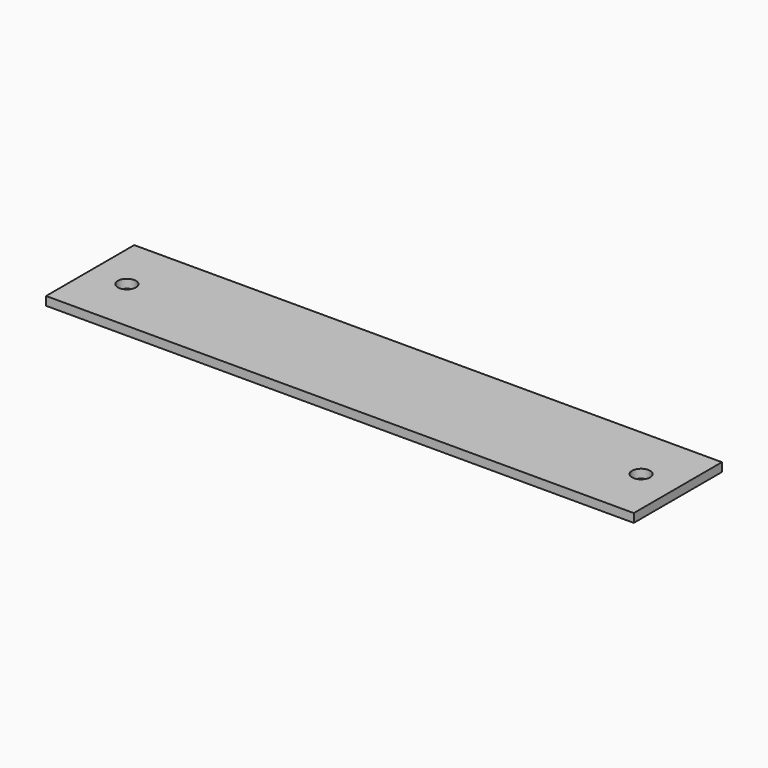
from build123d import *

# Parameters (mm, degrees)
F1_DEPTH = 3


with BuildPart() as f1:
    # F0 (on Top) → F1 (new body)
    with BuildSketch(Plane.XY):
        with BuildLine():
            Line((95.9196680397, 3.7129714398), (-5.6803319603, 3.7129714398))
            Line((-5.6803319603, 3.7129714398), (-5.6803319603, -15.3370285602))
            Line((-5.6803319603, -15.3370285602), (45.1196680397, -15.3370285602))
            Line((45.1196680397, -15.3370285602), (70.5196680397, -15.3370285602))
            Line((70.5196680397, -15.3370285602), (80.0952486641, -15.3370285602))
            ThreePointArc((80.0952486641, -15.3370285602), (83.2196680397, -12.2126091846), (86.3440874153, -15.3370285602))
            Line((86.3440874153, -15.3370285602), (95.9196680397, -15.3370285602))
            Line((95.9196680397, -15.3370285602), (95.9196680397, 3.7129714398))
        make_face()
        with BuildLine():
            Line((-97.7047513359, -15.3370285602), (-107.2803319603, -15.3370285602))
            Line((-107.2803319603, -15.3370285602), (-107.2803319603, -34.3870285602))
            Line((-107.2803319603, -34.3870285602), (-5.6803319603, -34.3870285602))
            Line((-5.6803319603, -34.3870285602), (-5.6803319603, -15.3370285602))
            Line((-5.6803319603, -15.3370285602), (-91.4559125847, -15.3370285602))
            ThreePointArc((-91.4559125847, -15.3370285602), (-94.5803319603, -18.4614479358), (-97.7047513359, -15.3370285602))
        make_face()
        with BuildLine():
            Line((45.1196680397, -15.3370285602), (-5.6803319603, -15.3370285602))
            Line((-5.6803319603, -15.3370285602), (-5.6803319603, -34.3870285602))
            Line((-5.6803319603, -34.3870285602), (95.9196680397, -34.3870285602))
            Line((95.9196680397, -34.3870285602), (95.9196680397, -15.3370285602))
            Line((95.9196680397, -15.3370285602), (86.3440874153, -15.3370285602))
            ThreePointArc((86.3440874153, -15.3370285602), (83.2196680397, -18.4614479358), (80.0952486641, -15.3370285602))
            Line((80.0952486641, -15.3370285602), (70.5196680397, -15.3370285602))
            Line((70.5196680397, -15.3370285602), (45.1196680397, -15.3370285602))
        make_face()
        with BuildLine():
            Line((-5.6803319603, 3.7129714398), (-107.2803319603, 3.7129714398))
            Line((-107.2803319603, 3.7129714398), (-107.2803319603, -15.3370285602))
            Line((-107.2803319603, -15.3370285602), (-97.7047513359, -15.3370285602))
            ThreePointArc((-97.7047513359, -15.3370285602), (-94.5803319603, -12.2126091846), (-91.4559125847, -15.3370285602))
            Line((-91.4559125847, -15.3370285602), (-5.6803319603, -15.3370285602))
            Line((-5.6803319603, -15.3370285602), (-5.6803319603, 3.7129714398))
        make_face()
    extrude(amount=F1_DEPTH)


solid = f1.part
